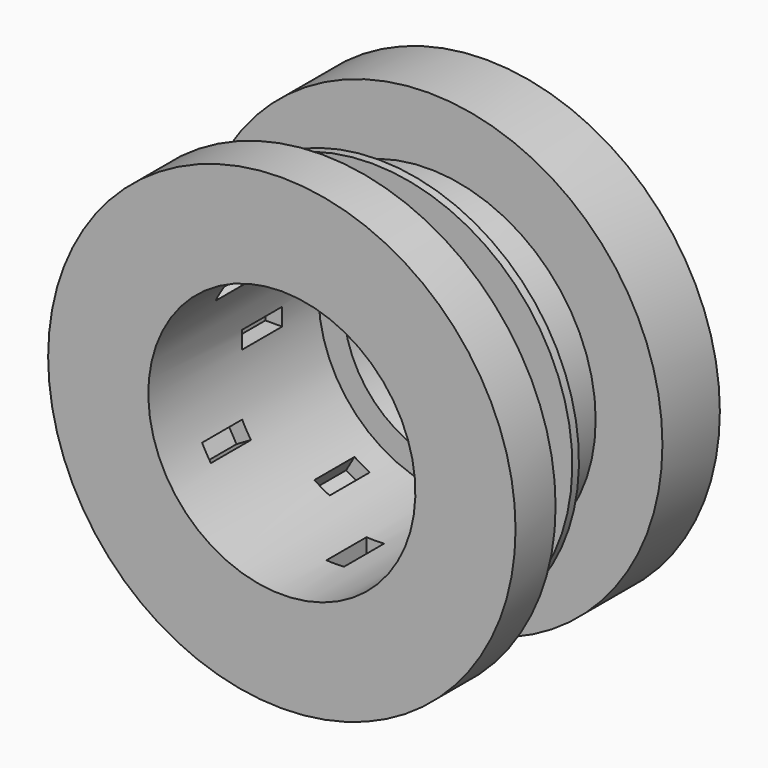
from build123d import *

# Parameters (mm, degrees)
F0_R            = 10
F0_R_2          = 8
F1_DEPTH        = 4
F3_DEPTH        = 3
F3_COPIES_COUNT = 3
F5_DEPTH        = 3
F5_COPIES_COUNT = 3
F7_DEPTH        = 3
F7_COPIES_COUNT = 3
F9_DEPTH        = 3
F9_COPIES_COUNT = 3
F10_W           = 0.5
F10_H           = 2
F10_W_2         = 3
F10_H_2         = 6


# Not quite as in the source:
# - a pattern or mirror of a feature is missing from the dataset's text; its kind, count and spacing are read off the source's solid


with BuildPart() as f1:
    # F0 (on Front) → F1 (new body, symmetric)
    with BuildSketch(Plane.XZ):
        Circle(F0_R)
        Circle(F0_R_2, mode=Mode.SUBTRACT)
    extrude(amount=F1_DEPTH, both=True)

    # F2 (on face) → F3 (cut)
    with BuildSketch(Plane.XZ.offset(4)):
        with BuildLine():
            Line((-0.525, 8.9827548503), (-0.525, 7.9827548503))
            ThreePointArc((-0.525, 7.9827548503), (0, 8), (0.525, 7.9827548503))
            Line((0.525, 7.9827548503), (0.525, 8.9827548503))
            Line((0.525, 8.9827548503), (-0.525, 8.9827548503))
        make_face()
    f3 = extrude(amount=-F3_DEPTH, mode=Mode.SUBTRACT)

    # F3_copies: F3 ×3 about axis
    f3_copies_axis = Axis((0, 0, 0), (0, 1, 0))
    for i in range(1, F3_COPIES_COUNT):
        add(f3.rotate(f3_copies_axis, i * 360 / F3_COPIES_COUNT), mode=Mode.SUBTRACT)

    # F4 (on Front) → F5 (cut)
    with BuildSketch(Plane.XZ):
        with BuildLine():
            ThreePointArc((6.6507684925, 4.4460407621), (6.9282032303, 4), (7.1757684925, 3.5367140882))
            Line((7.1757684925, 3.5367140882), (8.0417938963, 4.0367140882))
            Line((8.0417938963, 4.0367140882), (7.5167938963, 4.9460407621))
            Line((7.5167938963, 4.9460407621), (6.6507684925, 4.4460407621))
        make_face()
    f5 = extrude(amount=F5_DEPTH, mode=Mode.SUBTRACT)

    # F5_copies: F5 ×3 about axis
    f5_copies_axis = Axis((0, 0, 0), (0, 1, 0))
    for i in range(1, F5_COPIES_COUNT):
        add(f5.rotate(f5_copies_axis, i * 360 / F5_COPIES_COUNT), mode=Mode.SUBTRACT)

    # F6 (on face) → F7 (cut)
    with BuildSketch(Plane(origin=(0, 4, 0), x_dir=(-1, 0, 0), z_dir=(0, 1, 0))):
        with BuildLine():
            ThreePointArc((3.5367140882, 7.1757684925), (4, 6.9282032303), (4.4460407621, 6.6507684925))
            Line((4.4460407621, 6.6507684925), (4.9460407621, 7.5167938963))
            Line((4.9460407621, 7.5167938963), (4.0367140882, 8.0417938963))
            Line((4.0367140882, 8.0417938963), (3.5367140882, 7.1757684925))
        make_face()
    f7 = extrude(amount=-F7_DEPTH, mode=Mode.SUBTRACT)

    # F7_copies: F7 ×3 about axis
    f7_copies_axis = Axis((0, 0, 0), (0, 1, 0))
    for i in range(1, F7_COPIES_COUNT):
        add(f7.rotate(f7_copies_axis, i * 360 / F7_COPIES_COUNT), mode=Mode.SUBTRACT)

    # F8 (on Front) → F9 (cut)
    with BuildSketch(Plane.XZ):
        with BuildLine():
            ThreePointArc((-7.9827548503, -0.525), (-8, 0), (-7.9827548503, 0.525))
            Line((-7.9827548503, 0.525), (-8.9827548503, 0.525))
            Line((-8.9827548503, 0.525), (-8.9827548503, -0.525))
            Line((-8.9827548503, -0.525), (-7.9827548503, -0.525))
        make_face()
    f9 = extrude(amount=-F9_DEPTH, mode=Mode.SUBTRACT)

    # F9_copies: F9 ×3 about axis
    f9_copies_axis = Axis((0, 0, 0), (0, 1, 0))
    for i in range(1, F9_COPIES_COUNT):
        add(f9.rotate(f9_copies_axis, i * 360 / F9_COPIES_COUNT), mode=Mode.SUBTRACT)

    # F10 (on Right) → F11 (revolve)
    with BuildSketch(Plane.YZ):
        Polygon((4, 14), (4, 8), (5.75, 8), (5.75, 6.5), (11.5, 6.5), (11.5, 8), (8.3, 8), (8.3, 14), align=None)
        with Locations((0, 11)):
            Rectangle(F10_W, F10_H)
        with Locations((-5.5, 11)):
            Rectangle(F10_W_2, F10_H_2)
    revolve(axis=Axis((0, 0, 0), (0, -1, 0)))


solid = f1.part
